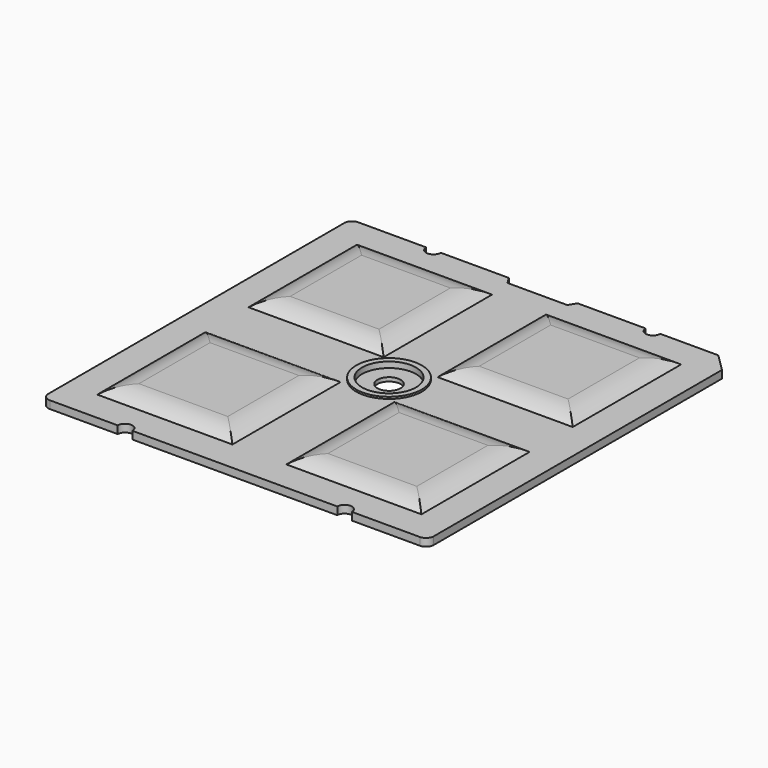
from build123d import *

# Parameters (mm, degrees)
F0_W         = 17.52
F0_H         = 17.52
F0_H_2       = 17.57
F0_R         = 1.5
F1_DEPTH     = 1
F2_W         = 17.52
F2_H         = 17.57
F2_H_2       = 17.52
F3_DEPTH     = 1
F4_R         = 3.5
F5_DEPTH     = 0.5
F6_R         = 4.25
F6_R_2       = 3.5
F7_DEPTH     = 0.25
F8_T1_DEPTH  = 32.52
F8_T3_DEPTH  = 32.52
F8_T5_DEPTH  = 32.57
F8_T7_DEPTH  = 32.52
F8_T12_DEPTH = 32.52
F8_S13_R     = 4.25
F8_T14_DEPTH = 18
F8_T18_DEPTH = 32.52
F8_S19_R     = 4.25
F8_T20_DEPTH = 18
F8_T24_DEPTH = 32.52
F8_S25_R     = 4.25
F8_T26_DEPTH = 18
F8_T30_DEPTH = 32.57
F8_S31_R     = 4.25
F8_T32_DEPTH = 18
F8_T36_DEPTH = 32.57
F8_S37_R     = 4.25
F8_T38_DEPTH = 18
F8_T42_DEPTH = 32.52
F8_S43_R     = 4.25
F8_T44_DEPTH = 18
F8_T48_DEPTH = 32.52
F8_S49_R     = 4.25
F8_T50_DEPTH = 18
F8_T54_DEPTH = 32.52
F8_S55_R     = 4.25
F8_T56_DEPTH = 18
F9_R         = 1.05
F10_DEPTH    = 0.5


# Not quite as in the source:
# - a fillet or chamfer that OpenCascade refuses, or shapes differently, is made with other operations: its cross-section is extruded or revolved along the edge and cut away or added


with BuildPart() as f1:
    # F0 (on Top) → F1 (new body)
    with BuildSketch(Plane.XY):
        with BuildLine():
            ThreePointArc((-25, -24), (-24.7071067812, -24.7071067812), (-24, -25))
            Line((-24, -25), (-15.1855654437, -25))
            ThreePointArc((-15.1855654437, -25), (-14.2350281943, -24.0494627506), (-13.2844909448, -25))
            Line((-13.2844909448, -25), (13.2844909448, -25))
            ThreePointArc((13.2844909448, -25), (14.2350281943, -24.0494627506), (15.1855654437, -25))
            Line((15.1855654437, -25), (24, -25))
            ThreePointArc((24, -25), (24.7071067812, -24.7071067812), (25, -24))
            Line((25, -24), (25, 22.7180756629))
            Line((25, 22.7180756629), (22.7180756629, 25))
            Line((22.7180756629, 25), (15.1855654437, 25))
            ThreePointArc((15.1855654437, 25), (14.2350281943, 24.0494627506), (13.2844909448, 25))
            Line((13.2844909448, 25), (4.4700563885, 25))
            Line((4.4700563885, 25), (3.8659917191, 24.0494627506))
            Line((3.8659917191, 24.0494627506), (0, 24.0494627506))
            Line((0, 24.0494627506), (-3.8659917191, 24.0494627506))
            Line((-3.8659917191, 24.0494627506), (-4.4700563885, 25))
            Line((-4.4700563885, 25), (-13.2844909448, 25))
            ThreePointArc((-13.2844909448, 25), (-14.2350281943, 24.0494627506), (-15.1855654437, 25))
            Line((-15.1855654437, 25), (-24, 25))
            ThreePointArc((-24, 25), (-24.7071067812, 24.7071067812), (-25, 24))
            Line((-25, 24), (-25, -24))
        make_face()
        with Locations((-12.26, -12.26)):
            Rectangle(F0_W, F0_H, mode=Mode.SUBTRACT)
        with Locations((12.26, -12.26)):
            Rectangle(F0_W, F0_H, mode=Mode.SUBTRACT)
        with Locations((-12.26, 12.285)):
            Rectangle(F0_W, F0_H_2, mode=Mode.SUBTRACT)
        Circle(F0_R, mode=Mode.SUBTRACT)
        with Locations((12.26, 12.285)):
            Rectangle(F0_W, F0_H_2, mode=Mode.SUBTRACT)
    extrude(amount=F1_DEPTH)

    # F2 (on face) → F3 (join, symmetric)
    with BuildSketch(Plane.XY.offset(1)):
        with Locations((-12.26, 12.285)):
            Rectangle(F2_W, F2_H)
        with Locations((12.26, 12.285)):
            Rectangle(F2_W, F2_H)
        with Locations((12.26, -12.26)):
            Rectangle(F2_W, F2_H_2)
        with Locations((-12.26, -12.26)):
            Rectangle(F2_W, F2_H_2)
    extrude(amount=F3_DEPTH, both=True)

    # F4 (on face) → F5 (cut)
    with BuildSketch(Plane.XY.offset(1)):
        Circle(F4_R)
    extrude(amount=-F5_DEPTH, mode=Mode.SUBTRACT)

    # F6 (on face) → F7 (join)
    with BuildSketch(Plane.XY.offset(1)):
        Circle(F6_R)
        Circle(F6_R_2, mode=Mode.SUBTRACT)
    extrude(amount=F7_DEPTH)

    # F8: fillet of radius 5 on 16 edges, made by hand

    # F8_s2 → F8_t1 (cut)
    with BuildSketch(Plane.YZ.offset(-28.52)):
        with BuildLine():
            ThreePointArc((-21.02, 1), (-19.6011388301, 1.7434164903), (-18.02, 2))
            Line((-18.02, 2), (-21.02, 2))
            Line((-21.02, 2), (-21.02, 1))
        make_face()
        with BuildLine():
            ThreePointArc((21.07, 1), (19.6511388301, 1.7434164903), (18.07, 2))
            Line((18.07, 2), (21.07, 2))
            Line((21.07, 2), (21.07, 1))
        make_face()
    extrude(amount=F8_T1_DEPTH, mode=Mode.SUBTRACT)

    # F8_s4 → F8_t3 (cut)
    with BuildSketch(Plane.XZ.offset(-4)):
        with BuildLine():
            ThreePointArc((-21.02, 1), (-19.6011388301, 1.7434164903), (-18.02, 2))
            Line((-18.02, 2), (-21.02, 2))
            Line((-21.02, 2), (-21.02, 1))
        make_face()
        with BuildLine():
            ThreePointArc((21.02, 1), (19.6011388301, 1.7434164903), (18.02, 2))
            Line((18.02, 2), (21.02, 2))
            Line((21.02, 2), (21.02, 1))
        make_face()
    extrude(amount=F8_T3_DEPTH, mode=Mode.SUBTRACT)

    # F8_s6 → F8_t5 (cut)
    with BuildSketch(Plane.XZ.offset(-28.57)):
        with BuildLine():
            ThreePointArc((-21.02, 1), (-19.6011388301, 1.7434164903), (-18.02, 2))
            Line((-18.02, 2), (-21.02, 2))
            Line((-21.02, 2), (-21.02, 1))
        make_face()
        with BuildLine():
            ThreePointArc((21.02, 1), (19.6011388301, 1.7434164903), (18.02, 2))
            Line((18.02, 2), (21.02, 2))
            Line((21.02, 2), (21.02, 1))
        make_face()
    extrude(amount=F8_T5_DEPTH, mode=Mode.SUBTRACT)

    # F8_s8 → F8_t7 (cut)
    with BuildSketch(Plane.YZ.offset(-4)):
        with BuildLine():
            ThreePointArc((21.07, 1), (19.6511388301, 1.7434164903), (18.07, 2))
            Line((18.07, 2), (21.07, 2))
            Line((21.07, 2), (21.07, 1))
        make_face()
        with BuildLine():
            ThreePointArc((-21.02, 1), (-19.6011388301, 1.7434164903), (-18.02, 2))
            Line((-18.02, 2), (-21.02, 2))
            Line((-21.02, 2), (-21.02, 1))
        make_face()
    extrude(amount=F8_T7_DEPTH, mode=Mode.SUBTRACT)


with BuildPart() as f8_tool10:
    # F8_s11 → F8_t12 (new body)
    with BuildSketch(Plane.XZ.offset(28.52)):
        with BuildLine():
            ThreePointArc((-3.5, 1), (-4.9188611699, 1.7434164903), (-6.5, 2))
            Line((-6.5, 2), (-3.5, 2))
            Line((-3.5, 2), (-3.5, 1))
        make_face()
    extrude(amount=-F8_T12_DEPTH)

    # F8_s13 → F8_t14 (cut, symmetric)
    with BuildSketch(Plane.XY.offset(1.5)):
        Circle(F8_S13_R)
    extrude(amount=F8_T14_DEPTH, both=True, mode=Mode.SUBTRACT)


with BuildPart() as f1_1:
    add(f1.part)

    # F8_t9: cut F8_tool10
    add(f8_tool10.part, mode=Mode.SUBTRACT)


with BuildPart() as f8_tool16:
    # F8_s17 → F8_t18 (new body)
    with BuildSketch(Plane.YZ.offset(4)):
        with BuildLine():
            ThreePointArc((-3.5, 1), (-4.9188611699, 1.7434164903), (-6.5, 2))
            Line((-6.5, 2), (-3.5, 2))
            Line((-3.5, 2), (-3.5, 1))
        make_face()
    extrude(amount=-F8_T18_DEPTH)

    # F8_s19 → F8_t20 (cut, symmetric)
    with BuildSketch(Plane.XY.offset(1.5)):
        Circle(F8_S19_R)
    extrude(amount=F8_T20_DEPTH, both=True, mode=Mode.SUBTRACT)


with BuildPart() as f1_2:
    add(f1_1.part)

    # F8_t15: cut F8_tool16
    add(f8_tool16.part, mode=Mode.SUBTRACT)


with BuildPart() as f8_tool22:
    # F8_s23 → F8_t24 (new body)
    with BuildSketch(Plane.YZ.offset(-28.52)):
        with BuildLine():
            ThreePointArc((3.5, 1), (4.9188611699, 1.7434164903), (6.5, 2))
            Line((6.5, 2), (3.5, 2))
            Line((3.5, 2), (3.5, 1))
        make_face()
    extrude(amount=F8_T24_DEPTH)

    # F8_s25 → F8_t26 (cut, symmetric)
    with BuildSketch(Plane.XY.offset(1.5)):
        Circle(F8_S25_R)
    extrude(amount=F8_T26_DEPTH, both=True, mode=Mode.SUBTRACT)


with BuildPart() as f1_3:
    add(f1_2.part)

    # F8_t21: cut F8_tool22
    add(f8_tool22.part, mode=Mode.SUBTRACT)


with BuildPart() as f8_tool28:
    # F8_s29 → F8_t30 (new body)
    with BuildSketch(Plane.XZ.offset(4)):
        with BuildLine():
            ThreePointArc((-3.5, 1), (-4.9188611699, 1.7434164903), (-6.5, 2))
            Line((-6.5, 2), (-3.5, 2))
            Line((-3.5, 2), (-3.5, 1))
        make_face()
    extrude(amount=-F8_T30_DEPTH)

    # F8_s31 → F8_t32 (cut, symmetric)
    with BuildSketch(Plane.XY.offset(1.5)):
        Circle(F8_S31_R)
    extrude(amount=F8_T32_DEPTH, both=True, mode=Mode.SUBTRACT)


with BuildPart() as f1_4:
    add(f1_3.part)

    # F8_t27: cut F8_tool28
    add(f8_tool28.part, mode=Mode.SUBTRACT)


with BuildPart() as f8_tool34:
    # F8_s35 → F8_t36 (new body)
    with BuildSketch(Plane.XZ.offset(-28.57)):
        with BuildLine():
            ThreePointArc((3.5, 1), (4.9188611699, 1.7434164903), (6.5, 2))
            Line((6.5, 2), (3.5, 2))
            Line((3.5, 2), (3.5, 1))
        make_face()
    extrude(amount=F8_T36_DEPTH)

    # F8_s37 → F8_t38 (cut, symmetric)
    with BuildSketch(Plane.XY.offset(1.5)):
        Circle(F8_S37_R)
    extrude(amount=F8_T38_DEPTH, both=True, mode=Mode.SUBTRACT)


with BuildPart() as f1_5:
    add(f1_4.part)

    # F8_t33: cut F8_tool34
    add(f8_tool34.part, mode=Mode.SUBTRACT)


with BuildPart() as f8_tool40:
    # F8_s41 → F8_t42 (new body)
    with BuildSketch(Plane.YZ.offset(-4)):
        with BuildLine():
            ThreePointArc((3.5, 1), (4.9188611699, 1.7434164903), (6.5, 2))
            Line((6.5, 2), (3.5, 2))
            Line((3.5, 2), (3.5, 1))
        make_face()
    extrude(amount=F8_T42_DEPTH)

    # F8_s43 → F8_t44 (cut, symmetric)
    with BuildSketch(Plane.XY.offset(1.5)):
        Circle(F8_S43_R)
    extrude(amount=F8_T44_DEPTH, both=True, mode=Mode.SUBTRACT)


with BuildPart() as f1_6:
    add(f1_5.part)

    # F8_t39: cut F8_tool40
    add(f8_tool40.part, mode=Mode.SUBTRACT)


with BuildPart() as f8_tool46:
    # F8_s47 → F8_t48 (new body)
    with BuildSketch(Plane.YZ.offset(28.52)):
        with BuildLine():
            ThreePointArc((-3.5, 1), (-4.9188611699, 1.7434164903), (-6.5, 2))
            Line((-6.5, 2), (-3.5, 2))
            Line((-3.5, 2), (-3.5, 1))
        make_face()
    extrude(amount=-F8_T48_DEPTH)

    # F8_s49 → F8_t50 (cut, symmetric)
    with BuildSketch(Plane.XY.offset(1.5)):
        Circle(F8_S49_R)
    extrude(amount=F8_T50_DEPTH, both=True, mode=Mode.SUBTRACT)


with BuildPart() as f1_7:
    add(f1_6.part)

    # F8_t45: cut F8_tool46
    add(f8_tool46.part, mode=Mode.SUBTRACT)


with BuildPart() as f8_tool52:
    # F8_s53 → F8_t54 (new body)
    with BuildSketch(Plane.XZ.offset(-4)):
        with BuildLine():
            ThreePointArc((3.5, 1), (4.9188611699, 1.7434164903), (6.5, 2))
            Line((6.5, 2), (3.5, 2))
            Line((3.5, 2), (3.5, 1))
        make_face()
    extrude(amount=F8_T54_DEPTH)

    # F8_s55 → F8_t56 (cut, symmetric)
    with BuildSketch(Plane.XY.offset(1.5)):
        Circle(F8_S55_R)
    extrude(amount=F8_T56_DEPTH, both=True, mode=Mode.SUBTRACT)


with BuildPart() as f1_8:
    add(f1_7.part)

    # F8_t51: cut F8_tool52
    add(f8_tool52.part, mode=Mode.SUBTRACT)

    # F9 (on face) → F10 (join)
    with BuildSketch(Plane(origin=(0, 0, 0), x_dir=(1, 0, 0), z_dir=(0, 0, -1))):
        with Locations((0, 22.5)):
            Circle(F9_R)
        with Locations((0, -22.5)):
            Circle(F9_R)
    extrude(amount=F10_DEPTH)


solid = f1_8.part
